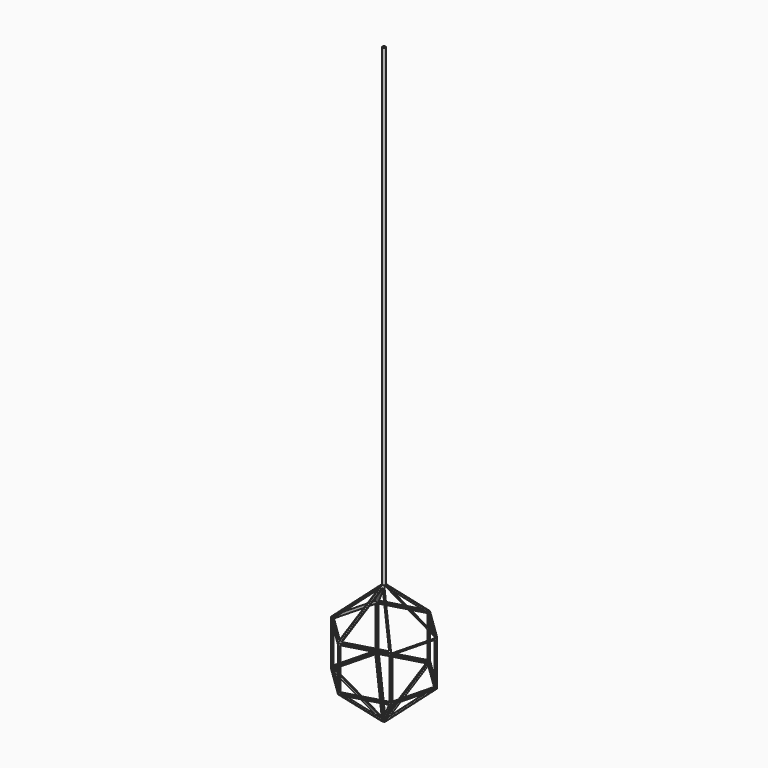
from build123d import *

# Parameters (mm, degrees)
F1_DEPTH  = 203.2
F2_SIZE   = 63.5
F3_T      = -2.54
F5_DEPTH  = 2.54
F7_DEPTH  = 2.54
F9_DEPTH  = 7.1852048969
F10_DEPTH = 2.541
F12_DEPTH = 2.54
F14_DEPTH = 2.54
F15_W     = 71.12
F15_H     = 71.12
F16_DEPTH = 157.0594794416
F17_W     = 71.12
F17_H     = 71.12
F18_DEPTH = 155.1690173594
F19_W     = 71.12
F19_H     = 71.12
F20_DEPTH = 170.067634702
F22_DEPTH = 2.54
F24_DEPTH = 2.54
F26_DEPTH = 2.54
F28_DEPTH = 2.54
F30_DEPTH = 2.54
F32_DEPTH = 2.54
F33_R     = 2.54
F34_DEPTH = 800


# Not quite as in the source:
# - a feature names something its author has since deleted; it is built from what else it names


with BuildPart() as f1:
    # F0 (on Top) → F1 (new body)
    with BuildSketch(Plane.XY):
        Polygon((73.3134762531, 20.774364002), (18.6656111534, 73.8785148759), (-54.6478650997, 53.104150874), (-73.3134762531, -20.774364002), (-18.6656111534, -73.8785148759), (54.6478650997, -53.104150874), align=None)
    extrude(amount=F1_DEPTH)

    # F2
    f2_edges = [f1.edges().sort_by_distance(p)[0] for p in [
        (45.989544, 47.326439, 203.2),
        (-17.991127, 63.491333, 203.2),
        (-63.980671, 16.164893, 203.2),
        (-45.989544, -47.326439, 203.2),
        (17.991127, -63.491333, 203.2),
        (63.980671, -16.164893, 203.2),
        (45.989544, 47.326439, 0),
        (-17.991127, 63.491333, 0),
        (-63.980671, 16.164893, 0),
        (-45.989544, -47.326439, 0),
        (17.991127, -63.491333, 0),
        (63.980671, -16.164893, 0),
    ]]
    chamfer(f2_edges, length=F2_SIZE)

    # F3
    f3_openings = [f1.faces().sort_by_distance(p)[0] for p in [
        (-42.712352, 10.791394, 161.636633),
    ]]
    offset(amount=F3_T, openings=f3_openings)

    # F4 (on face) → F5 (cut, through all)
    with BuildSketch(Plane(origin=(-71.6735768194, -73.7570960609, 102.8455678842), x_dir=(0.8701504485, -0.287188723, 0.4004507889), z_dir=(-0.4927861574, -0.5071112335, 0.7071067812))):
        Polygon((2.6696402664, 64.4858378393), (59.2408259088, 25.6139572621), (78.5633694658, 114.3351670347), align=None)
    extrude(amount=-F5_DEPTH, mode=Mode.SUBTRACT)

    # F6 (on face) → F7 (cut, through all)
    with BuildSketch(Plane(origin=(28.0387304884, -98.9496863361, 102.8455678842), x_dir=(0.9812423716, 0.1336581106, -0.1389205444), z_dir=(0.192778132, -0.6803209476, 0.7071067812))):
        Polygon((-44.3893807317, 46.8522479636), (22.9119959884, 60.3373077027), (-27.2544501276, 136.0217938087), align=None)
    extrude(amount=-F7_DEPTH, mode=Mode.SUBTRACT)

    # F8 (on face) → F9 (cut, through all)
    with BuildSketch(Plane(origin=(99.7123073078, -25.1925902753, 102.8455678842), x_dir=(0.7280120913, 0.1631104703, -0.6658778937), z_dir=(0.6855642894, -0.1732097142, 0.7071067812))):
        Polygon((-133.1636625665, 49.1073482105), (-134.131528973, 46.3985518281), (-61.9006782251, -18.3416021227), (-36.2615283041, 53.4154462512), align=None)
        Polygon((-63.0205602981, -13.9269250267), (-130.6368034196, 46.6771789529), (-39.925449456, 50.7100458165), align=None, mode=Mode.SUBTRACT)
    extrude(amount=-F9_DEPTH, mode=Mode.SUBTRACT)

    # F8 (on face) + F2_face2 (on face) → F10 (cut, through all)
    with BuildSketch(Plane(origin=(99.7123073078, -25.1925902753, 102.8455678842), x_dir=(0.7280120913, 0.1631104703, -0.6658778937), z_dir=(0.6855642894, -0.1732097142, 0.7071067812))):
        Polygon((-133.1636625665, 49.1073482105), (-134.131528973, 46.3985518281), (-61.9006782251, -18.3416021227), (-36.2615283041, 53.4154462512), align=None)
        Polygon((-63.0205602981, -13.9269250267), (-130.6368034196, 46.6771789529), (-39.925449456, 50.7100458165), align=None, mode=Mode.SUBTRACT)
    with BuildSketch(Plane(origin=(42.71235225, -10.7913939511, 161.636632955), x_dir=(0.2449555269, 0.969534316, 0), z_dir=(0.6855642894, -0.1732097142, 0.7071067812))):
        Polygon((-34.3195357799, -28.4830838377), (34.3195357799, -28.4830838377), (0, 55.5822670322), align=None)
    extrude(amount=-F10_DEPTH, mode=Mode.SUBTRACT)

    # F11 (on face) → F12 (cut, through all)
    with BuildSketch(Plane(origin=(71.6735768194, 73.7570960609, 102.8455678842), x_dir=(0.8701504485, -0.287188723, -0.4004507889), z_dir=(0.4927861574, 0.5071112335, 0.7071067812))):
        Polygon((-59.2408259088, -25.6139572621), (-78.5633694658, -114.3351670347), (-2.6696402664, -64.4858378393), align=None)
    extrude(amount=-F12_DEPTH, mode=Mode.SUBTRACT)

    # F13 (on face) → F14 (cut, through all)
    with BuildSketch(Plane(origin=(-28.0387304884, 98.9496863361, 102.8455678842), x_dir=(0.9812423716, 0.1336581106, 0.1389205444), z_dir=(-0.192778132, 0.6803209476, 0.7071067812))):
        Polygon((44.3893807317, -46.8522479636), (-22.9119959884, -60.3373077027), (27.2544501276, -136.0217938087), align=None)
    extrude(amount=-F14_DEPTH, mode=Mode.SUBTRACT)

    # F15 (on face) → F16 (cut, through all)
    with BuildSketch(Plane(origin=(17.9911269732, -63.4913328749, 0), x_dir=(0.9621191109, 0.2726294488, 0), z_dir=(0.2726294488, -0.9621191109, 0))):
        with Locations((0, 101.6)):
            Rectangle(F15_W, F15_H)
    extrude(amount=-F16_DEPTH, mode=Mode.SUBTRACT)

    # F17 (on face) → F18 (cut, through all)
    with BuildSketch(Plane(origin=(63.9806706764, -16.164893436, 0), x_dir=(0.2449555269, 0.969534316, 0), z_dir=(0.969534316, -0.2449555269, 0))):
        with Locations((0, 101.6)):
            Rectangle(F17_W, F17_H)
    extrude(amount=-F18_DEPTH, mode=Mode.SUBTRACT)

    # F19 (on face) → F20 (cut, through all)
    with BuildSketch(Plane(origin=(45.9895437032, 47.3264394389, 0), x_dir=(-0.717163584, 0.6969048671, 0), z_dir=(0.6969048671, 0.717163584, 0))):
        with Locations((0, 101.6)):
            Rectangle(F19_W, F19_H)
    extrude(amount=-F20_DEPTH, mode=Mode.SUBTRACT)

    # F21 (on face) → F22 (cut, through all)
    with BuildSketch(Plane(origin=(1.2076208066, -0.3051087374, -1.2455678842), x_dir=(0.7280120913, 0.1631104703, 0.6658778937), z_dir=(0.6855642894, -0.1732097142, -0.7071067812))):
        Polygon((95.3809385521, -2.3644010884), (72.2858277101, 62.2725697547), (4.6695845886, 1.6684657751), align=None)
    extrude(amount=-F22_DEPTH, mode=Mode.SUBTRACT)

    # F23 (on face) → F24 (cut, through all)
    with BuildSketch(Plane(origin=(0.8680423208, 0.8932759279, -1.2455678842), x_dir=(0.8701504485, -0.287188723, 0.4004507889), z_dir=(0.4927861574, 0.5071112335, -0.7071067812))):
        Polygon((22.13077439, -92.8080958564), (78.7019600324, -53.9362152793), (2.808230833, -4.0868860838), align=None)
    extrude(amount=-F24_DEPTH, mode=Mode.SUBTRACT)

    # F25 (on face) → F26 (cut, through all)
    with BuildSketch(Plane(origin=(-0.3395784858, 1.1983846653, -1.2455678842), x_dir=(0.9812423716, 0.1336581106, -0.1389205444), z_dir=(-0.192778132, 0.6803209476, -0.7071067812))):
        Polygon((16.1607261154, -94.0316157631), (-0.9742044888, -4.862069918), (-51.1406506047, -80.546556024), align=None)
    extrude(amount=-F26_DEPTH, mode=Mode.SUBTRACT)

    # F27 (on face) → F28 (cut, through all)
    with BuildSketch(Plane(origin=(-1.2076208066, 0.3051087374, -1.2455678842), x_dir=(0.7280120913, 0.1631104703, -0.6658778937), z_dir=(-0.6855642894, 0.1732097142, -0.7071067812))):
        Polygon((-72.2858277101, -62.2725697547), (-4.6695845886, -1.6684657751), (-95.3809385521, 2.3644010884), align=None)
    extrude(amount=-F28_DEPTH, mode=Mode.SUBTRACT)

    # F29 (on face) → F30 (cut, through all)
    with BuildSketch(Plane(origin=(-0.8680423208, -0.8932759279, -1.2455678842), x_dir=(0.8701504485, -0.287188723, -0.4004507889), z_dir=(-0.4927861574, -0.5071112335, -0.7071067812))):
        Polygon((-78.7019600324, 53.9362152793), (-2.808230833, 4.0868860838), (-22.13077439, 92.8080958564), align=None)
    extrude(amount=-F30_DEPTH, mode=Mode.SUBTRACT)

    # F31 (on face) → F32 (cut, through all)
    with BuildSketch(Plane(origin=(0.3395784858, -1.1983846653, -1.2455678842), x_dir=(0.9812423716, 0.1336581106, 0.1389205444), z_dir=(0.192778132, -0.6803209476, -0.7071067812))):
        Polygon((-16.1607261154, 94.0316157631), (0.9742044888, 4.862069918), (51.1406506047, 80.546556024), align=None)
    extrude(amount=-F32_DEPTH, mode=Mode.SUBTRACT)

    # F33 (on face) → F34 (join)
    with BuildSketch(Plane.XY.offset(203.2)):
        Circle(F33_R)
    extrude(amount=F34_DEPTH)


solid = f1.part
